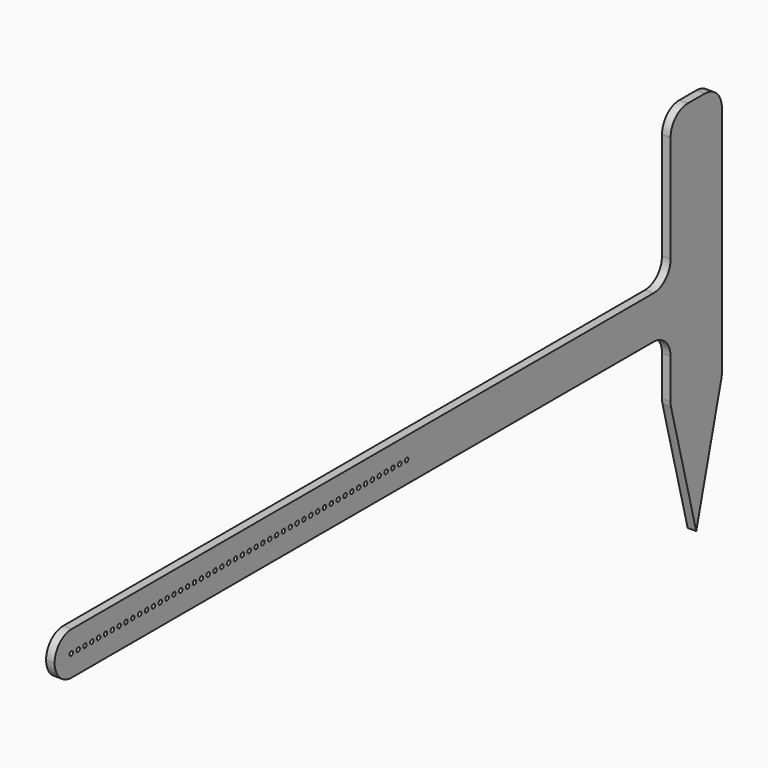
from build123d import *

# Parameters (mm, degrees)
F0_W     = 180
F0_H     = 10
F0_R     = 0.5
F1_DEPTH = 2
F2_R     = 4.99999


# Not quite as in the source:
# - a fillet or chamfer is up to 0.001 mm smaller than in the source, because OpenCascade refuses the exact size


with BuildPart() as f1:
    # F0 (on Right) → F1 (new body)
    with BuildSketch(Plane.YZ):
        Polygon((78.3572724922, 47.473322805), (78.3572724922, 12.473322805), (78.3572724922, 2.473322805), (78.3572724922, -12.526677195), (93.3572724922, -12.526677195), (93.3572724922, 47.473322805), align=None)
        with Locations((-11.6427275078, 7.473322805)):
            Rectangle(F0_W, F0_H)
        with Locations((-96.7759713531, 7.473322805)):
            Circle(F0_R, mode=Mode.SUBTRACT)
        with Locations((-94.7759713531, 7.473322805)):
            Circle(F0_R, mode=Mode.SUBTRACT)
        with Locations((-92.7759713531, 7.473322805)):
            Circle(F0_R, mode=Mode.SUBTRACT)
        with Locations((-90.7759713531, 7.473322805)):
            Circle(F0_R, mode=Mode.SUBTRACT)
        with Locations((-88.7759713531, 7.473322805)):
            Circle(F0_R, mode=Mode.SUBTRACT)
        with Locations((-86.7759713531, 7.473322805)):
            Circle(F0_R, mode=Mode.SUBTRACT)
        with Locations((-84.7759713531, 7.473322805)):
            Circle(F0_R, mode=Mode.SUBTRACT)
        with Locations((-82.7759713531, 7.473322805)):
            Circle(F0_R, mode=Mode.SUBTRACT)
        with Locations((-80.7759713531, 7.473322805)):
            Circle(F0_R, mode=Mode.SUBTRACT)
        with Locations((-78.7759713531, 7.473322805)):
            Circle(F0_R, mode=Mode.SUBTRACT)
        with Locations((-76.7759713531, 7.473322805)):
            Circle(F0_R, mode=Mode.SUBTRACT)
        with Locations((-74.7759713531, 7.473322805)):
            Circle(F0_R, mode=Mode.SUBTRACT)
        with Locations((-72.7759713531, 7.473322805)):
            Circle(F0_R, mode=Mode.SUBTRACT)
        with Locations((-70.7759713531, 7.473322805)):
            Circle(F0_R, mode=Mode.SUBTRACT)
        with Locations((-68.7759713531, 7.473322805)):
            Circle(F0_R, mode=Mode.SUBTRACT)
        with Locations((-66.7759713531, 7.473322805)):
            Circle(F0_R, mode=Mode.SUBTRACT)
        with Locations((-64.7759713531, 7.473322805)):
            Circle(F0_R, mode=Mode.SUBTRACT)
        with Locations((-62.7759713531, 7.473322805)):
            Circle(F0_R, mode=Mode.SUBTRACT)
        with Locations((-60.7759713531, 7.473322805)):
            Circle(F0_R, mode=Mode.SUBTRACT)
        with Locations((-58.7759713531, 7.473322805)):
            Circle(F0_R, mode=Mode.SUBTRACT)
        with Locations((-56.7759713531, 7.473322805)):
            Circle(F0_R, mode=Mode.SUBTRACT)
        with Locations((-54.7759713531, 7.473322805)):
            Circle(F0_R, mode=Mode.SUBTRACT)
        with Locations((-52.7759713531, 7.473322805)):
            Circle(F0_R, mode=Mode.SUBTRACT)
        with Locations((-50.7759713531, 7.473322805)):
            Circle(F0_R, mode=Mode.SUBTRACT)
        with Locations((-48.7759713531, 7.473322805)):
            Circle(F0_R, mode=Mode.SUBTRACT)
        with Locations((-46.7759713531, 7.473322805)):
            Circle(F0_R, mode=Mode.SUBTRACT)
        with Locations((-44.7759713531, 7.473322805)):
            Circle(F0_R, mode=Mode.SUBTRACT)
        with Locations((-42.7759713531, 7.473322805)):
            Circle(F0_R, mode=Mode.SUBTRACT)
        with Locations((-40.7759713531, 7.473322805)):
            Circle(F0_R, mode=Mode.SUBTRACT)
        with Locations((-38.7759713531, 7.473322805)):
            Circle(F0_R, mode=Mode.SUBTRACT)
        with Locations((-36.7759713531, 7.473322805)):
            Circle(F0_R, mode=Mode.SUBTRACT)
        with Locations((-34.7759713531, 7.473322805)):
            Circle(F0_R, mode=Mode.SUBTRACT)
        with Locations((-32.7759713531, 7.473322805)):
            Circle(F0_R, mode=Mode.SUBTRACT)
        with Locations((-30.7759713531, 7.473322805)):
            Circle(F0_R, mode=Mode.SUBTRACT)
        with Locations((-28.7759713531, 7.473322805)):
            Circle(F0_R, mode=Mode.SUBTRACT)
        with Locations((-26.7759713531, 7.473322805)):
            Circle(F0_R, mode=Mode.SUBTRACT)
        with Locations((-24.7759713531, 7.473322805)):
            Circle(F0_R, mode=Mode.SUBTRACT)
        with Locations((-22.7759713531, 7.473322805)):
            Circle(F0_R, mode=Mode.SUBTRACT)
        with Locations((-20.7759713531, 7.473322805)):
            Circle(F0_R, mode=Mode.SUBTRACT)
        with Locations((-18.7759713531, 7.473322805)):
            Circle(F0_R, mode=Mode.SUBTRACT)
        with Locations((-16.7759713531, 7.473322805)):
            Circle(F0_R, mode=Mode.SUBTRACT)
        with Locations((-14.7759713531, 7.473322805)):
            Circle(F0_R, mode=Mode.SUBTRACT)
        with Locations((-12.7759713531, 7.473322805)):
            Circle(F0_R, mode=Mode.SUBTRACT)
        with Locations((-10.7759713531, 7.473322805)):
            Circle(F0_R, mode=Mode.SUBTRACT)
        with Locations((-8.7759713531, 7.473322805)):
            Circle(F0_R, mode=Mode.SUBTRACT)
        with Locations((-6.7759713531, 7.473322805)):
            Circle(F0_R, mode=Mode.SUBTRACT)
        with Locations((-4.7759713531, 7.473322805)):
            Circle(F0_R, mode=Mode.SUBTRACT)
        with Locations((-2.7759713531, 7.473322805)):
            Circle(F0_R, mode=Mode.SUBTRACT)
        with Locations((-0.7759713531, 7.473322805)):
            Circle(F0_R, mode=Mode.SUBTRACT)
        with Locations((1.2240286469, 7.473322805)):
            Circle(F0_R, mode=Mode.SUBTRACT)
        Polygon((93.3572724922, -12.526677195), (78.3572724922, -12.526677195), (85.8572724922, -41.5740522915), align=None)
    extrude(amount=F1_DEPTH)

    # F2 (radius 5 in the source; OpenCascade refuses exactly that, so slightly less here)
    f2_edges = [f1.edges().sort_by_distance(p)[0] for p in [
        (1, 93.357272, 47.473323),
        (1, 78.357272, 47.473323),
        (1, 78.357272, 12.473323),
        (1, 78.357272, 2.473323),
        (1, 78.357272, -12.526677),
        (1, 93.357272, -12.526677),
        (1, -101.642728, 12.473323),
        (1, -101.642728, 2.473323),
    ]]
    fillet(f2_edges, radius=F2_R)


solid = f1.part
